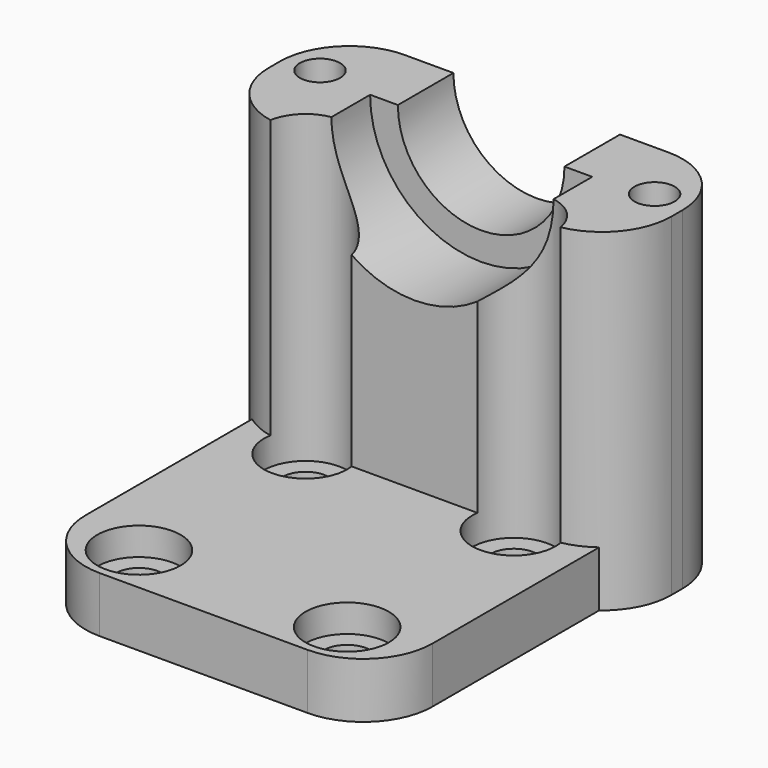
from build123d import *

# Parameters (mm, degrees)
F0_W          = 25
F0_H          = 30
F1_DEPTH      = 4
F2_R          = 1.675
F3_DEPTH      = 25
F4_W          = 25
F4_H          = 11
F5_DEPTH      = 20
F7_DEPTH      = 6
F8_R          = 8
F9_DEPTH      = 6
F2_R_2        = 3
F10_DEPTH     = 2
F11_W         = 11
F11_H         = 24
F12_DEPTH     = 2
F13_R         = 5
F14_W         = 11
F14_H         = 24
F15_DEPTH     = 2
F16_DEPTH     = 2
F17_R         = 1.45
F18_DEPTH     = 25
F19_T1_DEPTH  = 49
F19_T6_DEPTH  = 49
F19_T11_DEPTH = 49
F19_T16_DEPTH = 49
F19_T21_DEPTH = 49
F20_DEPTH     = 25


# Not quite as in the source:
# - a fillet or chamfer that OpenCascade refuses, or shapes differently, is made with other operations: its cross-section is extruded or revolved along the edge and cut away or added


with BuildPart() as f1:
    # F0 (on Top) → F1 (new body)
    with BuildSketch(Plane.XY):
        with Locations((12.5, 15)):
            Rectangle(F0_W, F0_H)
    extrude(amount=F1_DEPTH)

    # F2 (on face) → F3 (cut)
    with BuildSketch(Plane.XY.offset(4)):
        with BuildLine():
            ThreePointArc((3.325, 18.5605346784), (5, 16.8855346784), (6.675, 18.5605346784))
            ThreePointArc((6.675, 18.5605346784), (5, 20.2355346784), (3.325, 18.5605346784))
        make_face()
        with Locations((20, 18.5605346784)):
            Circle(F2_R)
        with Locations((20, 3.5605346784)):
            Circle(F2_R)
        with Locations((5, 3.5605346784)):
            Circle(F2_R)
    extrude(amount=-F3_DEPTH, mode=Mode.SUBTRACT)

    # F4 (on face) → F5 (join)
    with BuildSketch(Plane.XY.offset(4)):
        with Locations((12.5, 24.5)):
            Rectangle(F4_W, F4_H)
    extrude(amount=F5_DEPTH)

    # F6 (on face) → F7 (cut)
    with BuildSketch(Plane(origin=(0, 30, 0), x_dir=(-1, 0, 0), z_dir=(0, 1, 0))):
        with BuildLine():
            ThreePointArc((-18.5, 24), (-12.5, 18), (-6.5, 24))
            Line((-6.5, 24), (-18.5, 24))
        make_face()
    extrude(amount=-F7_DEPTH, mode=Mode.SUBTRACT)

    # F8 (on face) → F9 (cut)
    with BuildSketch(Plane.XZ.offset(-19)):
        with Locations((12.5, 24)):
            Circle(F8_R)
    extrude(amount=-F9_DEPTH, mode=Mode.SUBTRACT)

    # F2 (on face) → F10 (cut)
    with BuildSketch(Plane.XY.offset(4)):
        with BuildLine():
            ThreePointArc((8, 18.5605346784), (5, 21.5605346784), (2, 18.5605346784))
            ThreePointArc((2, 18.5605346784), (5, 15.5605346784), (8, 18.5605346784))
        make_face()
        with BuildLine():
            ThreePointArc((3.325, 18.5605346784), (5, 20.2355346784), (6.675, 18.5605346784))
            ThreePointArc((6.675, 18.5605346784), (5, 16.8855346784), (3.325, 18.5605346784))
        make_face(mode=Mode.SUBTRACT)
        with Locations((20, 18.5605346784)):
            Circle(F2_R_2)
        with Locations((20, 18.5605346784)):
            Circle(F2_R, mode=Mode.SUBTRACT)
        with Locations((20, 3.5605346784)):
            Circle(F2_R_2)
        with Locations((20, 3.5605346784)):
            Circle(F2_R, mode=Mode.SUBTRACT)
        with Locations((5, 3.5605346784)):
            Circle(F2_R_2)
        with Locations((5, 3.5605346784)):
            Circle(F2_R, mode=Mode.SUBTRACT)
    extrude(amount=-F10_DEPTH, mode=Mode.SUBTRACT)

    # F11 (on face) → F12 (join)
    with BuildSketch(Plane(origin=(0, 0, 0), x_dir=(0, -1, 0), z_dir=(-1, 0, 0))):
        with Locations((-24.5, 12)):
            Rectangle(F11_W, F11_H)
    extrude(amount=F12_DEPTH)

    # F13
    f13_edges = [f1.edges().sort_by_distance(p)[0] for p in [
        (0, 0, 2),
        (25, 0, 2),
    ]]
    fillet(f13_edges, radius=F13_R)

    # F14 (on face) → F15 (join)
    with BuildSketch(Plane.YZ.offset(25)):
        with Locations((24.5, 12)):
            Rectangle(F14_W, F14_H)
    extrude(amount=F15_DEPTH)

    # F14 (on face) → F16 (join)
    with BuildSketch(Plane.YZ.offset(25)):
        with Locations((24.5, 12)):
            Rectangle(F14_W, F14_H)
    extrude(amount=F16_DEPTH)

    # F17 (on face) → F18 (cut)
    with BuildSketch(Plane.XY.offset(24)):
        with Locations((0.45, 25.55)):
            Circle(F17_R)
        with Locations((24.55, 25.55)):
            Circle(F17_R)
    extrude(amount=-F18_DEPTH, mode=Mode.SUBTRACT)

    # F19: fillet of radius 5 on 4 edges, made by hand

    # F19_s2 → F19_t1 (cut)
    with BuildSketch(Plane.XY.offset(-12.5)):
        with BuildLine():
            ThreePointArc((-2, 25), (-0.5355339059, 28.5355339059), (3, 30))
            Line((3, 30), (-2, 30))
            Line((-2, 30), (-2, 25))
        make_face()
        with BuildLine():
            ThreePointArc((22, 30), (25.5355339059, 28.5355339059), (27, 25))
            Line((27, 25), (27, 30))
            Line((27, 30), (22, 30))
        make_face()
    extrude(amount=F19_T1_DEPTH, mode=Mode.SUBTRACT)


with BuildPart() as f19_tool4:
    # F19_s5 → F19_t6 (new body)
    with BuildSketch(Plane.XY.offset(-12.5)):
        with BuildLine():
            ThreePointArc((3, 19), (-0.5355339059, 20.4644660941), (-2, 24))
            Line((-2, 24), (-2, 19))
            Line((-2, 19), (3, 19))
        make_face()
    extrude(amount=F19_T6_DEPTH)

    split(bisect_by=Plane.YZ, keep=Keep.BOTTOM)


with BuildPart() as f1_1:
    add(f1.part)

    # F19_t3: cut F19_tool4
    add(f19_tool4.part, mode=Mode.SUBTRACT)


with BuildPart() as f19_tool9:
    # F19_s10 → F19_t11 (new body)
    with BuildSketch(Plane.XY.offset(-12.5)):
        with BuildLine():
            ThreePointArc((3, 19), (-0.5355339059, 20.4644660941), (-2, 24))
            Line((-2, 24), (-2, 19))
            Line((-2, 19), (3, 19))
        make_face()
    extrude(amount=F19_T11_DEPTH)

    split(bisect_by=Plane.XY.offset(4), keep=Keep.TOP)


with BuildPart() as f1_2:
    add(f1_1.part)

    # F19_t8: cut F19_tool9
    add(f19_tool9.part, mode=Mode.SUBTRACT)


with BuildPart() as f19_tool14:
    # F19_s15 → F19_t16 (new body)
    with BuildSketch(Plane.XY.offset(36.5)):
        with BuildLine():
            ThreePointArc((22, 19), (25.5355339059, 20.4644660941), (27, 24))
            Line((27, 24), (27, 19))
            Line((27, 19), (22, 19))
        make_face()
    extrude(amount=-F19_T16_DEPTH)

    split(bisect_by=Plane.XY.offset(4), keep=Keep.TOP)


with BuildPart() as f1_3:
    add(f1_2.part)

    # F19_t13: cut F19_tool14
    add(f19_tool14.part, mode=Mode.SUBTRACT)


with BuildPart() as f19_tool19:
    # F19_s20 → F19_t21 (new body)
    with BuildSketch(Plane.XY.offset(36.5)):
        with BuildLine():
            ThreePointArc((22, 19), (25.5355339059, 20.4644660941), (27, 24))
            Line((27, 24), (27, 19))
            Line((27, 19), (22, 19))
        make_face()
    extrude(amount=-F19_T21_DEPTH)

    split(bisect_by=Plane.YZ.offset(25), keep=Keep.TOP)


with BuildPart() as f1_4:
    add(f1_3.part)

    # F19_t18: cut F19_tool19
    add(f19_tool19.part, mode=Mode.SUBTRACT)

    # F2 (on face) → F20 (cut)
    with BuildSketch(Plane.XY.offset(4)):
        with BuildLine():
            ThreePointArc((8, 18.5605346784), (5, 21.5605346784), (2, 18.5605346784))
            ThreePointArc((2, 18.5605346784), (5, 15.5605346784), (8, 18.5605346784))
        make_face()
        with BuildLine():
            ThreePointArc((3.325, 18.5605346784), (5, 20.2355346784), (6.675, 18.5605346784))
            ThreePointArc((6.675, 18.5605346784), (5, 16.8855346784), (3.325, 18.5605346784))
        make_face(mode=Mode.SUBTRACT)
        with Locations((20, 18.5605346784)):
            Circle(F2_R_2)
        with Locations((20, 18.5605346784)):
            Circle(F2_R, mode=Mode.SUBTRACT)
        with BuildLine():
            ThreePointArc((3.325, 18.5605346784), (5, 16.8855346784), (6.675, 18.5605346784))
            ThreePointArc((6.675, 18.5605346784), (5, 20.2355346784), (3.325, 18.5605346784))
        make_face()
        with Locations((20, 18.5605346784)):
            Circle(F2_R)
    extrude(amount=F20_DEPTH, mode=Mode.SUBTRACT)


solid = f1_4.part
